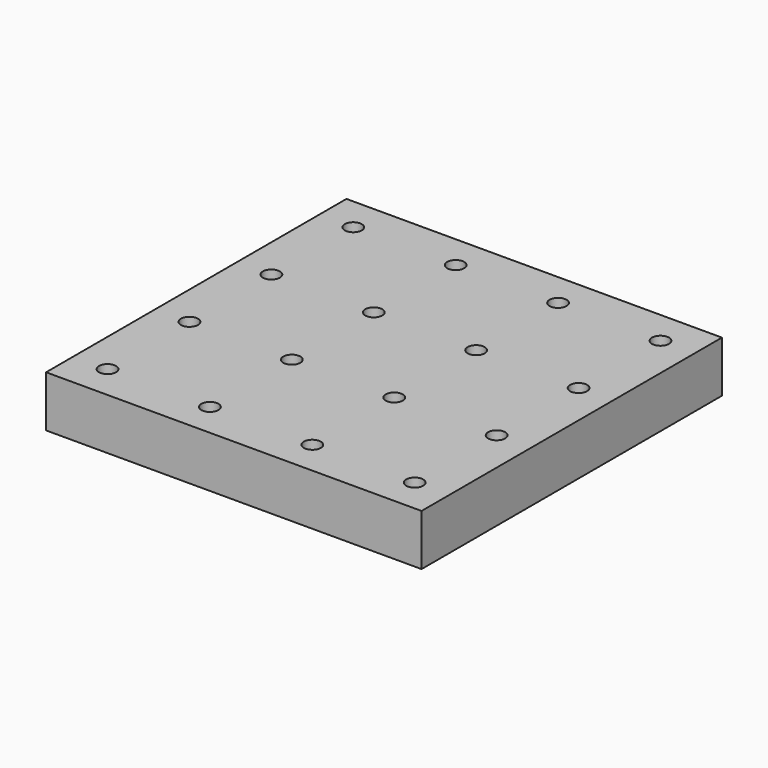
from build123d import *

# Parameters (mm, degrees)
F0_W     = 110
F0_H     = 110
F0_R     = 2.5
F1_DEPTH = 15


# Not quite as in the source:
# - the program builds the solid bodies; features that only make, move or delete a surface that nothing else refers to are left out


with BuildPart() as f1:
    # F0 (on Top) → F1 (new body)
    with BuildSketch(Plane.XY):
        Rectangle(F0_W, F0_H)
        with Locations((-45, -45)):
            Circle(F0_R, mode=Mode.SUBTRACT)
        with Locations((-15, -45)):
            Circle(F0_R, mode=Mode.SUBTRACT)
        with Locations((-45, -15)):
            Circle(F0_R, mode=Mode.SUBTRACT)
        with Locations((-15, -15)):
            Circle(F0_R, mode=Mode.SUBTRACT)
        with Locations((15, -45)):
            Circle(F0_R, mode=Mode.SUBTRACT)
        with Locations((45, -45)):
            Circle(F0_R, mode=Mode.SUBTRACT)
        with Locations((15, -15)):
            Circle(F0_R, mode=Mode.SUBTRACT)
        with Locations((45, -15)):
            Circle(F0_R, mode=Mode.SUBTRACT)
        with Locations((-45, 15)):
            Circle(F0_R, mode=Mode.SUBTRACT)
        with Locations((-15, 15)):
            Circle(F0_R, mode=Mode.SUBTRACT)
        with Locations((-45, 45)):
            Circle(F0_R, mode=Mode.SUBTRACT)
        with Locations((-15, 45)):
            Circle(F0_R, mode=Mode.SUBTRACT)
        with Locations((15, 15)):
            Circle(F0_R, mode=Mode.SUBTRACT)
        with Locations((45, 15)):
            Circle(F0_R, mode=Mode.SUBTRACT)
        with Locations((15, 45)):
            Circle(F0_R, mode=Mode.SUBTRACT)
        with Locations((45, 45)):
            Circle(F0_R, mode=Mode.SUBTRACT)
    extrude(amount=F1_DEPTH)


solid = f1.part
